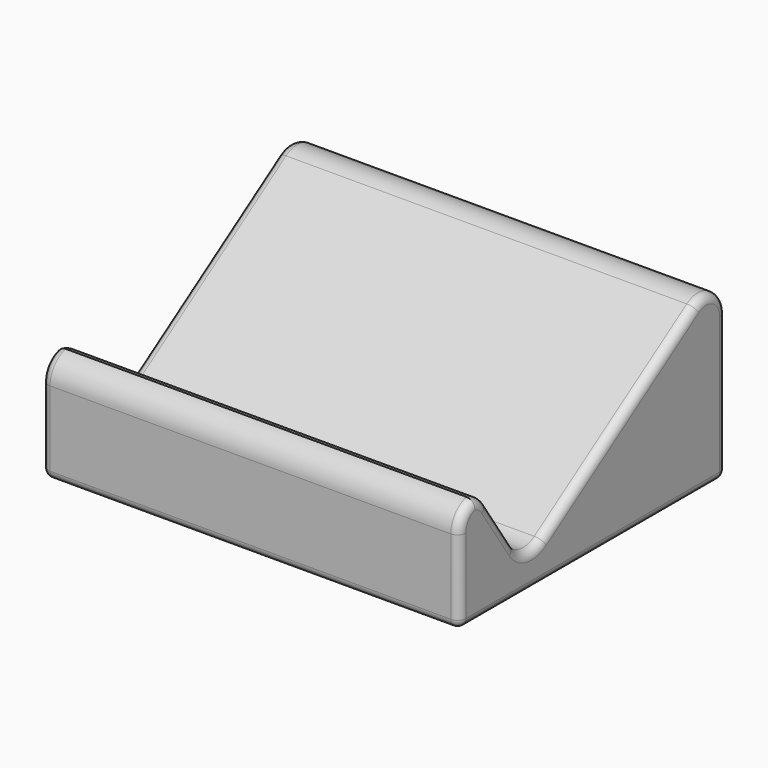
from build123d import *

# Parameters (mm, degrees)
F0_W         = 50
F0_H         = 40
F1_DEPTH     = 3
F2_W         = 50
F2_H         = 30
F3_DEPTH     = 20
F5_DEPTH     = 50
F6_W         = 50
F6_H         = 10
F7_DEPTH     = 10
F9_DEPTH     = 50
F10_T1_DEPTH = 50
F10_T3_DEPTH = 58.0277563773
F10_T5_DEPTH = 65
F10_T7_DEPTH = 78.0277563773
F11_R        = 1


# Not quite as in the source:
# - a fillet or chamfer that OpenCascade refuses, or shapes differently, is made with other operations: its cross-section is extruded or revolved along the edge and cut away or added


with BuildPart() as f1:
    # F0 (on Top) → F1 (new body)
    with BuildSketch(Plane.XY):
        Rectangle(F0_W, F0_H)
    extrude(amount=F1_DEPTH)

    # F2 (on face) → F3 (join)
    with BuildSketch(Plane.XY.offset(3)):
        with Locations((0, 5)):
            Rectangle(F2_W, F2_H)
    extrude(amount=F3_DEPTH)

    # F4 (on face) → F5 (cut, through all)
    with BuildSketch(Plane.YZ.offset(25)):
        Polygon((-10, 23), (-10, 3), (20, 23), align=None)
    extrude(amount=-F5_DEPTH, mode=Mode.SUBTRACT)

    # F6 (on face) → F7 (join)
    with BuildSketch(Plane.XY.offset(3)):
        with Locations((0, -15)):
            Rectangle(F6_W, F6_H)
    extrude(amount=F7_DEPTH)

    # F8 (on face) → F9 (cut, through all)
    with BuildSketch(Plane.YZ.offset(25)):
        Polygon((-16.6666666667, 13), (-10, 3), (-10, 13), align=None)
    extrude(amount=-F9_DEPTH, mode=Mode.SUBTRACT)

    # F10: fillet of radius 3 on 4 edges, made by hand

    # F10_s2 → F10_t1 (join)
    with BuildSketch(Plane.YZ.offset(-25)):
        with BuildLine():
            ThreePointArc((-11.6641005887, 5.496150883), (-9.7562981111, 4.2185094446), (-7.503849117, 4.6641005887))
            Line((-7.503849117, 4.6641005887), (-10, 3))
            Line((-10, 3), (-11.6641005887, 5.496150883))
        make_face()
    extrude(amount=F10_T1_DEPTH)

    # F10_s4 → F10_t3 (cut)
    with BuildSketch(Plane.YZ.offset(-29.0138781887)):
        with BuildLine():
            ThreePointArc((-18.2722179421, 13), (-16.8566441655, 12.6450237963), (-15.7760670591, 11.6641005887))
            Line((-15.7760670591, 11.6641005887), (-16.6666666667, 13))
            Line((-16.6666666667, 13), (-18.2722179421, 13))
        make_face()
    extrude(amount=F10_T3_DEPTH, mode=Mode.SUBTRACT)

    # F10_s6 → F10_t5 (cut)
    with BuildSketch(Plane.YZ.offset(-32.5)):
        with BuildLine():
            ThreePointArc((-20, 10), (-19.1213203436, 12.1213203436), (-17, 13))
            Line((-17, 13), (-20, 13))
            Line((-20, 13), (-20, 10))
        make_face()
    extrude(amount=F10_T5_DEPTH, mode=Mode.SUBTRACT)

    # F10_s8 → F10_t7 (cut)
    with BuildSketch(Plane.YZ.offset(-39.0138781887)):
        with BuildLine():
            ThreePointArc((20, 17.3944487245), (18.4155737766, 20.0394725208), (15.3358994113, 19.8905996075))
            Line((15.3358994113, 19.8905996075), (20, 23))
            Line((20, 23), (20, 17.3944487245))
        make_face()
    extrude(amount=F10_T7_DEPTH, mode=Mode.SUBTRACT)

    # F11
    f11_edges = [f1.edges().sort_by_distance(p)[0] for p in [
        (25, 3.916025, 12.27735),
        (-25, 3.916025, 12.27735),
        (-25, -20, 5),
        (25, -20, 5),
        (25, 0, 0),
        (0, 20, 0),
        (-25, 0, 0),
        (0, -20, 0),
        (-25, 20, 8.697224),
        (-25, -19.335415, 11.883039),
        (-25, -16.582686, 12.479008),
        (-25, -13.720084, 8.580126),
        (-25, -9.756298, 4.218509),
        (-25, 18.415574, 20.039473),
        (25, 20, 8.697224),
        (25, 18.415574, 20.039473),
        (25, -9.756298, 4.218509),
        (25, -13.720084, 8.580126),
        (25, -16.582686, 12.479008),
        (25, -19.335415, 11.883039),
    ]]
    fillet(f11_edges, radius=F11_R)


solid = f1.part
